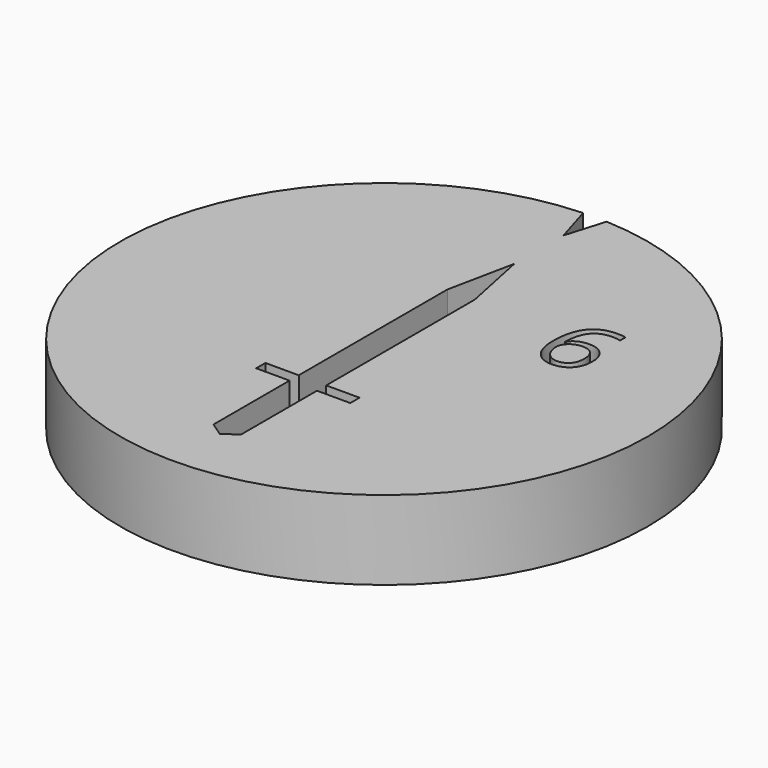
from build123d import *

# Parameters (mm, degrees)
F0_R         = 12.7
F1_DEPTH     = 3.81
F2_TEXT_SIZE = 4.7455557958
F3_DEPTH     = 2.54


# Not quite as in the source:
# - Text() gives the source's letters only with a copy of the font that has no kerning and outlines rounded to 1/6400 em; it was checked with that copy


with BuildPart() as f1:
    # F0 (on Top) → F1 (new body)
    with BuildSketch(Plane.XY):
        Circle(F0_R)
    extrude(amount=F1_DEPTH)

    # F2 (on face) → F3 (cut)
    with BuildSketch(Plane.XY.offset(3.81)):
        Polygon((2.2655467119, -4.8595412585), (2.2655467119, -4.3033502947), (0.6604, -4.3033502947), (0.6604, 4.6348046739), (0, 7.8382246), (-0.6604, 4.6348046739), (-0.6604, -4.3033502947), (-2.2655467119, -4.3033502947), (-2.2655467119, -4.8595412585), (-0.6604, -4.8595412585), (-0.6604, -9.4300005933), (0, -9.8820896819), (0.6604, -9.4300005933), (0.6604, -4.8595412585), align=None)
        with Locations((4.7818296589, 2.3815997411)):
            Text('6', F2_TEXT_SIZE, font='Open Sans', text_align=(TextAlign.LEFT, TextAlign.BOTTOM))
        with BuildLine():
            ThreePointArc((0.563748814, 12.6874815182), (0, 12.7), (-0.563748814, 12.6874815182))
            Line((-0.563748814, 12.6874815182), (0, 10.795))
            Line((0, 10.795), (0.563748814, 12.6874815182))
        make_face()
    extrude(amount=-F3_DEPTH, mode=Mode.SUBTRACT)


solid = f1.part
